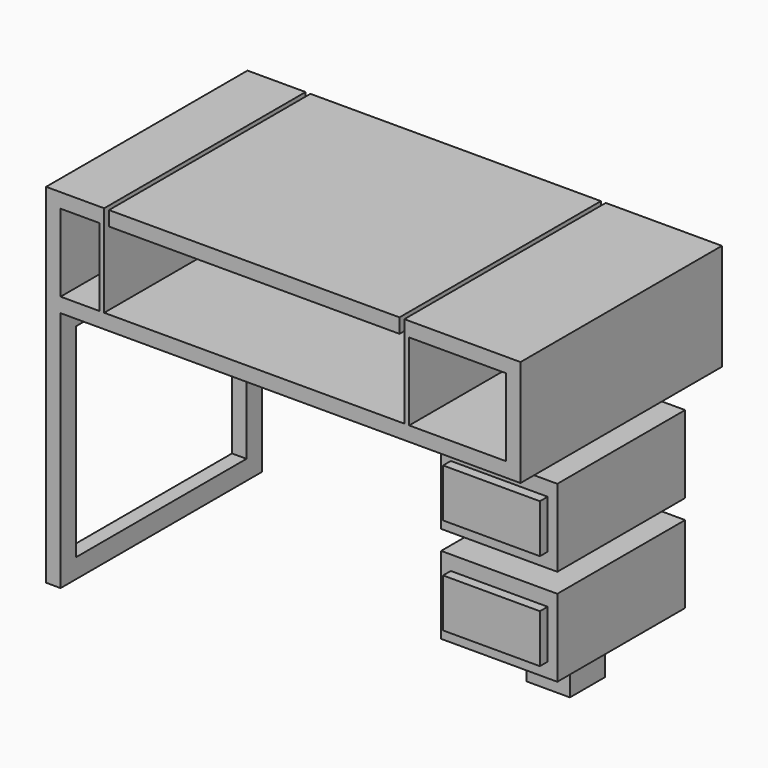
from build123d import *

# Parameters (mm, degrees)
F0_W      = 12.7
F0_H      = 203.2
F1_DEPTH  = 660.4
F0_W_2    = 762
F0_H_2    = 38.1
F3_W      = 558.8
F3_H      = 533.4
F4_DEPTH  = 38.1
F6_W      = 114.3
F6_H      = 114.3
F7_DEPTH  = 635
F8_W      = 419.1
F8_H      = 203.2
F9_DEPTH  = 304.8
F10_W     = 254
F10_H     = 127
F11_DEPTH = 25.4
F12_DEPTH = 406.4
F13_W     = 25.4
F13_H     = 203.2
F14_DEPTH = 101.6
F15_R     = 101.59999
F17_W     = 762
F17_H     = 76.2
F18_DEPTH = 25.4
F16_R     = 6.35
F19_DEPTH = 609.6
F20_DEPTH = 152.4


# Not quite as in the source:
# - a fillet or chamfer is up to 0.001 mm smaller than in the source, because OpenCascade refuses the exact size


with BuildPart() as f1:
    # F0 (on Front) → F1 (new body)
    with BuildSketch(Plane.XZ):
        Polygon((-63.6245734215, 386.4844668388), (-63.6245734215, 424.5844668388), (-216.0245734215, 424.5844668388), (-216.0245734215, 386.4844668388), (-209.6745734215, 386.4844668388), (-209.6745734215, 399.1844668388), (-196.9745734215, 399.1844668388), (-196.9745734215, 386.4844668388), (-190.6245734215, 386.4844668388), (-190.6245734215, 399.1844668388), (-177.9245734215, 399.1844668388), (-177.9245734215, 386.4844668388), (-76.3245734215, 386.4844668388), align=None)
        with Locations((-69.9745734215, 284.8844668388)):
            Rectangle(F0_W, F0_H)
        Polygon((-209.6745734215, 386.4844668388), (-216.0245734215, 386.4844668388), (-216.0245734215, -489.8155331612), (-177.9245734215, -489.8155331612), (-177.9245734215, 145.1844668388), (-177.9245734215, 183.2844668388), (-177.9245734215, 221.3844668388), (-177.9245734215, 386.4844668388), (-177.9245734215, 399.1844668388), (-190.6245734215, 399.1844668388), (-190.6245734215, 386.4844668388), (-196.9745734215, 386.4844668388), (-196.9745734215, 399.1844668388), (-209.6745734215, 399.1844668388), align=None)
        Polygon((723.7754265785, 183.2844668388), (-63.6245734215, 183.2844668388), (-76.3245734215, 183.2844668388), (-177.9245734215, 183.2844668388), (-177.9245734215, 145.1844668388), (990.4754265785, 145.1844668388), (990.4754265785, 183.2844668388), (736.4754265785, 183.2844668388), align=None)
        with Locations((730.1254265785, 284.8844668388)):
            Rectangle(F0_W, F0_H)
        Polygon((723.7754265785, 424.5844668388), (723.7754265785, 386.4844668388), (736.4754265785, 386.4844668388), (990.4754265785, 386.4844668388), (990.4754265785, 399.1844668388), (1003.1754265785, 399.1844668388), (1003.1754265785, 386.4844668388), (1009.5254265785, 386.4844668388), (1009.5254265785, 399.1844668388), (1022.2254265785, 399.1844668388), (1022.2254265785, 386.4844668388), (1028.5754265785, 386.4844668388), (1028.5754265785, 424.5844668388), align=None)
        Polygon((990.4754265785, 386.4844668388), (990.4754265785, 183.2844668388), (990.4754265785, 145.1844668388), (1028.5754265785, 145.1844668388), (1028.5754265785, 386.4844668388), (1022.2254265785, 386.4844668388), (1022.2254265785, 399.1844668388), (1009.5254265785, 399.1844668388), (1009.5254265785, 386.4844668388), (1003.1754265785, 386.4844668388), (1003.1754265785, 399.1844668388), (990.4754265785, 399.1844668388), align=None)
    extrude(amount=-F1_DEPTH)

    # F3 (on face) → F4 (cut)
    with BuildSketch(Plane(origin=(-216.0245734215, 0, 0), x_dir=(0, -1, 0), z_dir=(-1, 0, 0))):
        with Locations((-330.2, -172.3155331612)):
            Rectangle(F3_W, F3_H)
    extrude(amount=-F4_DEPTH, mode=Mode.SUBTRACT)

    # F6 (on face) → F7 (join)
    with BuildSketch(Plane(origin=(0, 0, 145.1844668388), x_dir=(1, 0, 0), z_dir=(0, 0, -1))):
        with Locations((882.5254265785, -330.2)):
            Rectangle(F6_W, F6_H)
    extrude(amount=F7_DEPTH)

    # F8 (on face) → F9 (join)
    with BuildSketch(Plane.YZ.offset(1028.5754265785)):
        with Locations((330.2, -7.2155331612)):
            Rectangle(F8_W, F8_H)
        with Locations((330.2, -261.2155331612)):
            Rectangle(F8_W, F8_H)
    extrude(amount=-F9_DEPTH)

    # F10 (on face) → F11 (join)
    with BuildSketch(Plane.XZ.offset(-120.65)):
        with Locations((876.1754265785, -7.2155331612)):
            Rectangle(F10_W, F10_H)
        with Locations((876.1754265785, -261.2155331612)):
            Rectangle(F10_W, F10_H)
    extrude(amount=F11_DEPTH)

    # F10 (on face) → F12 (cut)
    with BuildSketch(Plane.XZ.offset(-120.65)):
        with Locations((876.1754265785, -7.2155331612)):
            Rectangle(F10_W, F10_H)
        with Locations((876.1754265785, -261.2155331612)):
            Rectangle(F10_W, F10_H)
    extrude(amount=-F12_DEPTH, mode=Mode.SUBTRACT)


with BuildPart() as f1b:
    # F0 (on Front) → F1, piece 2 (new body)
    with BuildSketch(Plane.XZ):
        with Locations((330.0754265785, 405.5344668388)):
            Rectangle(F0_W_2, F0_H_2)
    extrude(amount=-F1_DEPTH)

    # F13 (on face) → F14 (join)
    with BuildSketch(Plane(origin=(0, 0, 386.4844668388), x_dir=(1, 0, 0), z_dir=(0, 0, -1))):
        with Locations((114.1754265785, -330.2)):
            Rectangle(F13_W, F13_H)
        with Locations((545.9754265785, -330.2)):
            Rectangle(F13_W, F13_H)
    extrude(amount=F14_DEPTH)

    # F15 (radius 101.6 in the source; OpenCascade refuses exactly that, so slightly less here)
    f15_edges = [f1b.edges().sort_by_distance(p)[0] for p in [
        (545.975427, 228.6, 284.884467),
        (545.975427, 431.8, 284.884467),
        (114.175427, 228.6, 284.884467),
        (114.175427, 431.8, 284.884467),
    ]]
    fillet(f15_edges, radius=F15_R)

    # F17 (on face) → F18 (join)
    with BuildSketch(Plane(origin=(0, 0, 386.4844668388), x_dir=(1, 0, 0), z_dir=(0, 0, -1))):
        with Locations((330.0754265785, -330.2)):
            Rectangle(F17_W, F17_H)
    extrude(amount=F18_DEPTH)

    # F16 (on face) → F19 (cut)
    with BuildSketch(Plane(origin=(101.4754265785, 0, 0), x_dir=(0, -1, 0), z_dir=(-1, 0, 0))):
        with BuildLine():
            Line((-393.7, 386.4844668388), (-406.4, 386.4844668388))
            ThreePointArc((-406.4, 386.4844668388), (-330.2, 310.2844668388), (-254, 386.4844668388))
            Line((-254, 386.4844668388), (-266.7, 386.4844668388))
            ThreePointArc((-266.7, 386.4844668388), (-330.2, 322.9844668388), (-393.7, 386.4844668388))
        make_face()
        with Locations((-330.2, 386.4844668388)):
            Circle(F16_R)
    extrude(amount=-F19_DEPTH, mode=Mode.SUBTRACT)

    # F16 (on face) → F20 (cut)
    with BuildSketch(Plane(origin=(101.4754265785, 0, 0), x_dir=(0, -1, 0), z_dir=(-1, 0, 0))):
        with BuildLine():
            Line((-393.7, 386.4844668388), (-406.4, 386.4844668388))
            ThreePointArc((-406.4, 386.4844668388), (-330.2, 310.2844668388), (-254, 386.4844668388))
            Line((-254, 386.4844668388), (-266.7, 386.4844668388))
            ThreePointArc((-266.7, 386.4844668388), (-330.2, 322.9844668388), (-393.7, 386.4844668388))
        make_face()
        with Locations((-330.2, 386.4844668388)):
            Circle(F16_R)
    extrude(amount=F20_DEPTH, mode=Mode.SUBTRACT)


with BuildPart() as f21_1:
    # F21: copy of F1b
    add(f1b.part)


solid = Compound([f1.part, f1b.part, f21_1.part])
